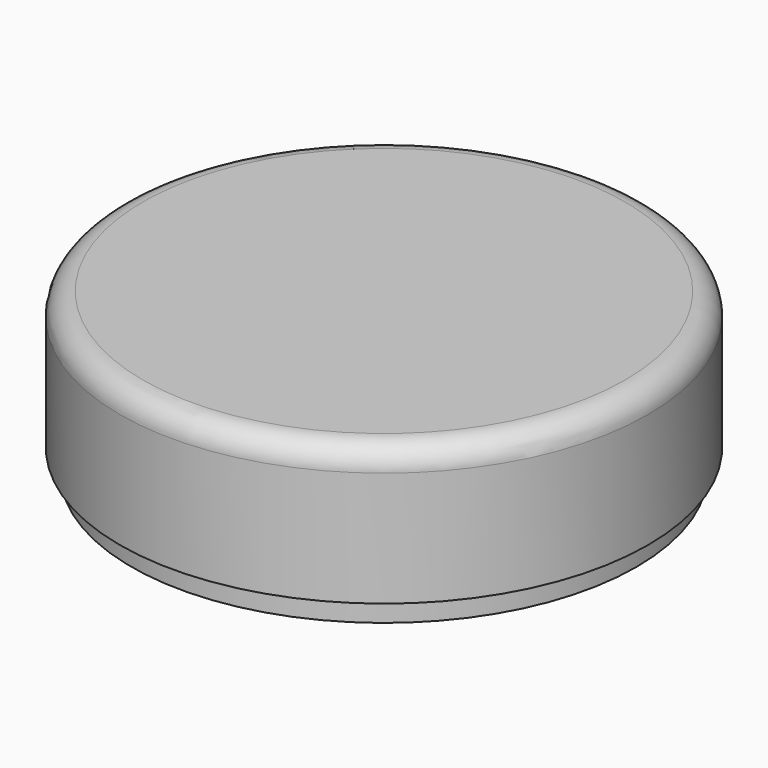
from build123d import *

# Parameters (mm, degrees)
F0_R     = 115
F1_DEPTH = 70
F2_R     = 17.5
F3_DEPTH = 7
F5_R     = 10
F6_R     = 115
F6_R_2   = 110
F7_DEPTH = 10


# Not quite as in the source:
# - a fillet or chamfer that OpenCascade refuses, or shapes differently, is made with other operations: its cross-section is extruded or revolved along the edge and cut away or added


with BuildPart() as f1:
    # F0 (on Top) → F1 (new body)
    with BuildSketch(Plane.XY):
        Circle(F0_R)
    extrude(amount=F1_DEPTH)

    # F2 (on face) → F3 (cut)
    with BuildSketch(Plane(origin=(0, 0, 0), x_dir=(1, 0, 0), z_dir=(0, 0, -1))):
        with Locations((-60, 60)):
            Circle(F2_R)
        with Locations((-60, -60)):
            Circle(F2_R)
        with Locations((60, -60)):
            Circle(F2_R)
        with Locations((60, 60)):
            Circle(F2_R)
    extrude(amount=-F3_DEPTH, mode=Mode.SUBTRACT)

    # F4: fillet of radius 12 on 4 edges, made by hand

    # F4_s1 → F4_t2 (revolve)
    with BuildSketch(Plane.XZ.offset(60)):
        with BuildLine():
            ThreePointArc((-42.5, 0), (-46.9279714162, 5.0995049384), (-53.4087121146, 7))
            Line((-53.4087121146, 7), (-42.5, 7))
            Line((-42.5, 7), (-42.5, 0))
        make_face()
    revolve(axis=Axis((-60, -60, 7), (0, 0, -1)))

    # F4_s3 → F4_t4 (revolve)
    with BuildSketch(Plane.XZ.offset(-60)):
        with BuildLine():
            ThreePointArc((-42.5, 0), (-46.9279714162, 5.0995049384), (-53.4087121146, 7))
            Line((-53.4087121146, 7), (-42.5, 7))
            Line((-42.5, 7), (-42.5, 0))
        make_face()
    revolve(axis=Axis((-60, 60, 7), (0, 0, -1)))

    # F4_s5 → F4_t6 (revolve)
    with BuildSketch(Plane.XZ.offset(-60)):
        with BuildLine():
            ThreePointArc((77.5, 0), (73.0720285838, 5.0995049384), (66.5912878854, 7))
            Line((66.5912878854, 7), (77.5, 7))
            Line((77.5, 7), (77.5, 0))
        make_face()
    revolve(axis=Axis((60, 60, 7), (0, 0, -1)))

    # F4_s7 → F4_t8 (revolve)
    with BuildSketch(Plane.XZ.offset(60)):
        with BuildLine():
            ThreePointArc((77.5, 0), (73.0720285838, 5.0995049384), (66.5912878854, 7))
            Line((66.5912878854, 7), (77.5, 7))
            Line((77.5, 7), (77.5, 0))
        make_face()
    revolve(axis=Axis((60, -60, 7), (0, 0, -1)))

    # F5
    f5_edges = [f1.edges().sort_by_distance(p)[0] for p in [
        (-115, 0, 70),
    ]]
    fillet(f5_edges, radius=F5_R)

    # F6 (on face) → F7 (cut)
    with BuildSketch(Plane(origin=(0, 0, 0), x_dir=(1, 0, 0), z_dir=(0, 0, -1))):
        Circle(F6_R)
        Circle(F6_R_2, mode=Mode.SUBTRACT)
    extrude(amount=-F7_DEPTH, mode=Mode.SUBTRACT)


solid = f1.part
